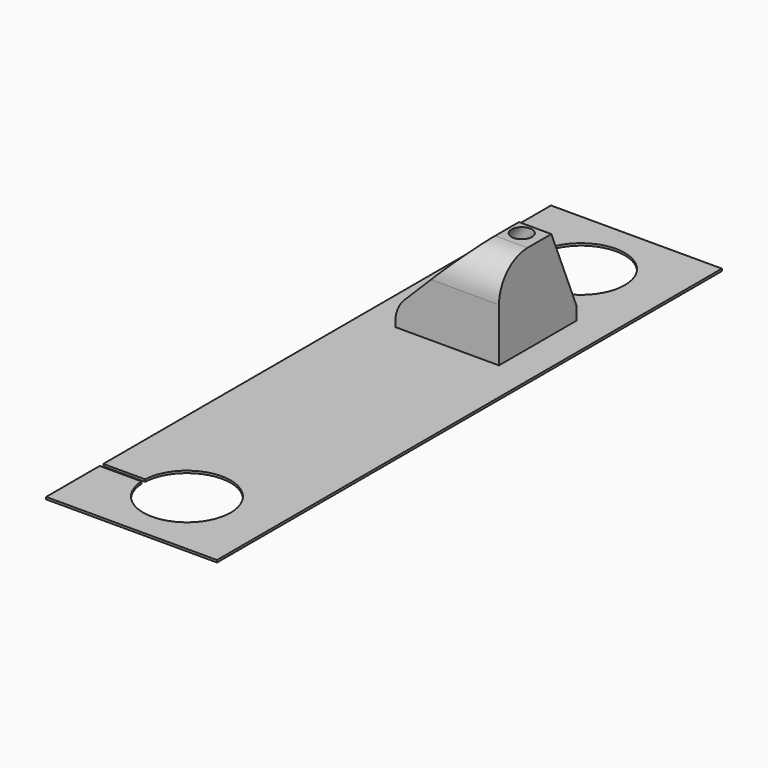
from build123d import *

# Parameters (mm, degrees)
F1_DEPTH     = 0.5
F2_W         = 23.2733339071
F2_H         = 21.7338502407
F3_DEPTH     = 20
F6_R         = 2.3033864012
F5_R         = 2.4232405009
F8_SIZE      = 16
F9_R         = 8
F10_R        = 7
F11_SIZE     = 7
F12_T1_DEPTH = 66.1267417653


# Not quite as in the source:
# - a fillet or chamfer that OpenCascade refuses, or shapes differently, is made with other operations: its cross-section is extruded or revolved along the edge and cut away or added


with BuildPart() as f1:
    # F0 (on Top) → F1 (new body)
    with BuildSketch(Plane.XY):
        with BuildLine():
            Line((19.1950201988, 70.8673447371), (-19.1950201988, 70.8673447371))
            Line((-19.1950201988, 70.8673447371), (-19.1950201988, 55.8184058152))
            Line((-19.1950201988, 55.8184058152), (-9.8077457496, 55.8184058152))
            ThreePointArc((-9.8077457496, 55.8184058152), (9.8204918965, 55.3182214499), (-9.8077457496, 54.8180370845))
            Line((-9.8077457496, 54.8180370845), (-19.1950201988, 54.8180370845))
            Line((-19.1950201988, 54.8180370845), (-19.1950201988, -54.8180370845))
            Line((-19.1950201988, -54.8180370845), (-9.8077457496, -54.8180370845))
            ThreePointArc((-9.8077457496, -54.8180370845), (9.8204918965, -55.3182214499), (-9.8077457496, -55.8184058152))
            Line((-9.8077457496, -55.8184058152), (-19.1950201988, -55.8184058152))
            Line((-19.1950201988, -55.8184058152), (-19.1950201988, -70.8673447371))
            Line((-19.1950201988, -70.8673447371), (19.1950201988, -70.8673447371))
            Line((19.1950201988, -70.8673447371), (19.1950201988, 70.8673447371))
        make_face()
    extrude(amount=F1_DEPTH)

    # F2 (on face) → F3 (join)
    with BuildSketch(Plane.XY.offset(0.5)):
        with Locations((0, 28.6038741469)):
            Rectangle(F2_W, F2_H)
    extrude(amount=F3_DEPTH)

    # F6 (on face) → F7 section 0
    with BuildSketch(Plane.XY.offset(20.5)):
        with Locations((7.3801875114, 29.4457376003)):
            Circle(F6_R)
    # F5 (on offset) → F7 section 1
    with BuildSketch(Plane.XY.offset(0.5)):
        with Locations((-7.0039108396, 29.0047153831)):
            Circle(F5_R)
    loft(mode=Mode.SUBTRACT)

    # F8
    f8_edges = [f1.edges().sort_by_distance(p)[0] for p in [
        (-11.636667, 28.603874, 20.5),
    ]]
    chamfer(f8_edges, length=F8_SIZE)

    # F9
    f9_edges = [f1.edges().sort_by_distance(p)[0] for p in [
        (8, 17.736949, 20.5),
    ]]
    fillet(f9_edges, radius=F9_R)

    # F10
    f10_edges = [f1.edges().sort_by_distance(p)[0] for p in [
        (-11.636667, 28.603874, 4.5),
    ]]
    fillet(f10_edges, radius=F10_R)

    # F11
    f11_edges = [f1.edges().sort_by_distance(p)[0] for p in [
        (8, 39.470799, 20.5),
    ]]
    chamfer(f11_edges, length=F11_SIZE)

    # F12: chamfer of 10 on 1 edges, made by hand

    # F12_s2 → F12_t1 (cut)
    with BuildSketch(Plane.YZ.offset(-28.5633708826)):
        Polygon((39.4707992673, 3.5), (32.3997314554, 20.5710678119), (39.4707992673, 13.5), align=None)
    extrude(amount=F12_T1_DEPTH, mode=Mode.SUBTRACT)


solid = f1.part
